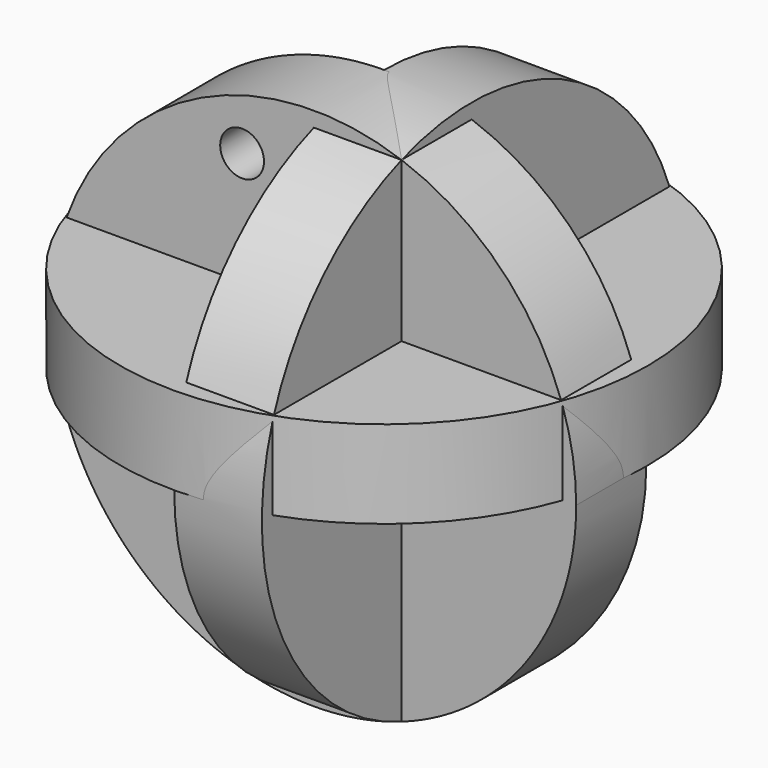
from build123d import *

# Parameters (mm, degrees)
F0_R     = 75.9892747742
F1_DEPTH = 25.4
F2_R     = 75.972189553
F3_DEPTH = 25.4
F4_R     = 76.4406104517
F5_DEPTH = 25.4
F7_D     = 12.7


with BuildPart() as f1:
    # F0 (on Front) → F1 (new body)
    with BuildSketch(Plane.XZ):
        Circle(F0_R)
    extrude(amount=F1_DEPTH)

    # F2 (on Right) → F3 (join)
    with BuildSketch(Plane.YZ):
        Circle(F2_R)
    extrude(amount=F3_DEPTH)

    # F4 (on Top) → F5 (join)
    with BuildSketch(Plane.XY):
        Circle(F4_R)
    extrude(amount=F5_DEPTH)

    # F7 (through all)
    with Locations(Plane(origin=(0, 0, 0), x_dir=(1, 0, 0), z_dir=(0, 1, 0))):
        with Locations((-20.7811314613, -58.2467317581)):
            Hole(F7_D / 2)


solid = f1.part
